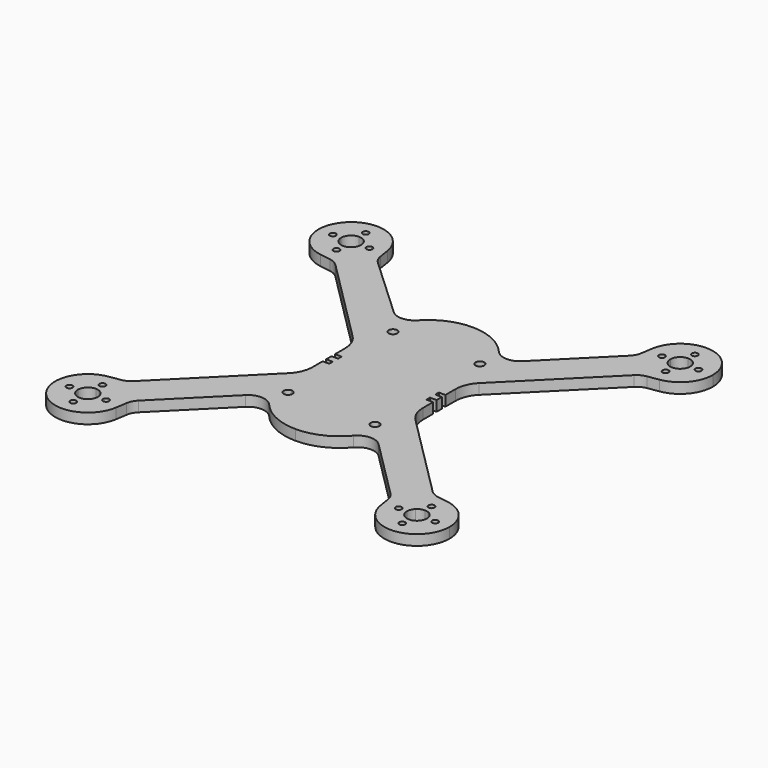
from build123d import *

# Parameters (mm, degrees)
F0_W     = 20
F0_H     = 20
F1_DEPTH = 2.38125


with BuildPart() as f1:
    # F0 (on Top) → F1 (new body)
    with BuildSketch(Plane.XY):
        with BuildLine():
            ThreePointArc((14.5598719395, -9.1717182668), (13.1833649686, -7.1116300018), (12.7, -4.6815902063))
            Line((12.7, -4.6815902063), (12.7, -1.778))
            Line((12.7, -1.778), (11.176, -1.778))
            Line((11.176, -1.778), (11.176, -0.762))
            Line((11.176, -0.762), (12.7, -0.762))
            Line((12.7, -0.762), (12.7, 0))
            Line((12.7, 0), (12.7, 0.762))
            Line((12.7, 0.762), (11.176, 0.762))
            Line((11.176, 0.762), (11.176, 1.778))
            Line((11.176, 1.778), (12.7, 1.778))
            Line((12.7, 1.778), (12.7, 4.6815902063))
            ThreePointArc((12.7, 4.6815902063), (13.1833649686, 7.1116300018), (14.5598719395, 9.1717182668))
            Line((14.5598719395, 9.1717182668), (34.3565237507, 28.9683700781))
            ThreePointArc((34.3565237507, 28.9683700781), (35.3250117586, 29.6711216441), (36.4637071746, 30.0388192574))
            Line((36.4637071746, 30.0388192574), (39.0000191321, 30.4342328562))
            ThreePointArc((39.0000191321, 30.4342328562), (35.5184477773, 30.7146069816), (32.5414162801, 32.5414162801))
            ThreePointArc((32.5414162801, 32.5414162801), (30.7146069816, 35.5184477773), (30.4342328562, 39.0000191321))
            Line((30.4342328562, 39.0000191321), (30.0388192574, 36.4637071746))
            ThreePointArc((30.0388192574, 36.4637071746), (29.6711216441, 35.3250117586), (28.9683700781, 34.3565237507))
            Line((28.9683700781, 34.3565237507), (15.290565472, 20.6787191446))
            ThreePointArc((15.290565472, 20.6787191446), (12.4394024333, 19.5660356884), (9.6896066428, 20.9098430623))
            ThreePointArc((9.6896066428, 20.9098430623), (5.3397094073, 24.2229121079), (0, 25.4))
            ThreePointArc((0, 25.4), (-5.0707891759, 24.3437578613), (-9.2981167449, 21.350723958))
            ThreePointArc((-9.2981167449, 21.350723958), (-11.9482165642, 20.1384898061), (-14.6798334501, 21.1537778832))
            Line((-14.6798334501, 21.1537778832), (-28.8786970448, 34.3361925702))
            ThreePointArc((-28.8786970448, 34.3361925702), (-29.650647044, 35.3400479178), (-30.0509413788, 36.5414624199))
            Line((-30.0509413788, 36.5414624199), (-30.4342328562, 39.0000191321))
            ThreePointArc((-30.4342328562, 39.0000191321), (-30.3671295561, 38.4240995168), (-30.344717139, 37.844717139))
            ThreePointArc((-30.344717139, 37.844717139), (-30.9156206452, 34.9745913963), (-32.5414162801, 32.5414162801))
            ThreePointArc((-32.5414162801, 32.5414162801), (-35.5184477773, 30.7146069816), (-39.0000191321, 30.4342328562))
            Line((-39.0000191321, 30.4342328562), (-36.4637071746, 30.0388192574))
            ThreePointArc((-36.4637071746, 30.0388192574), (-35.3250117586, 29.6711216441), (-34.3565237507, 28.9683700781))
            Line((-34.3565237507, 28.9683700781), (-14.5598719395, 9.1717182668))
            ThreePointArc((-14.5598719395, 9.1717182668), (-13.1833649686, 7.1116300018), (-12.7, 4.6815902063))
            Line((-12.7, 4.6815902063), (-12.7, 1.778))
            Line((-12.7, 1.778), (-11.176, 1.778))
            Line((-11.176, 1.778), (-11.176, 0.762))
            Line((-11.176, 0.762), (-12.7, 0.762))
            Line((-12.7, 0.762), (-12.7, 0))
            Line((-12.7, 0), (-12.7, -0.762))
            Line((-12.7, -0.762), (-11.176, -0.762))
            Line((-11.176, -0.762), (-11.176, -1.778))
            Line((-11.176, -1.778), (-12.7, -1.778))
            Line((-12.7, -1.778), (-12.7, -4.6815902063))
            ThreePointArc((-12.7, -4.6815902063), (-13.1833649686, -7.1116300018), (-14.5598719395, -9.1717182668))
            Line((-14.5598719395, -9.1717182668), (-34.3565237507, -28.9683700781))
            ThreePointArc((-34.3565237507, -28.9683700781), (-35.3250117586, -29.6711216441), (-36.4637071746, -30.0388192574))
            Line((-36.4637071746, -30.0388192574), (-39.0000191321, -30.4342328562))
            ThreePointArc((-39.0000191321, -30.4342328562), (-35.5184477773, -30.7146069816), (-32.5414162801, -32.5414162801))
            ThreePointArc((-32.5414162801, -32.5414162801), (-30.9156206452, -34.9745913963), (-30.344717139, -37.844717139))
            ThreePointArc((-30.344717139, -37.844717139), (-30.3671295561, -38.4240995168), (-30.4342328562, -39.0000191321))
            Line((-30.4342328562, -39.0000191321), (-30.0388192574, -36.4637071746))
            ThreePointArc((-30.0388192574, -36.4637071746), (-29.6711216441, -35.3250117586), (-28.9683700781, -34.3565237507))
            Line((-28.9683700781, -34.3565237507), (-15.290565472, -20.6787191446))
            ThreePointArc((-15.290565472, -20.6787191446), (-12.4394024333, -19.5660356884), (-9.6896066428, -20.9098430623))
            ThreePointArc((-9.6896066428, -20.9098430623), (-5.3397094073, -24.2229121079), (0, -25.4))
            ThreePointArc((0, -25.4), (5.3397094073, -24.2229121079), (9.6896066428, -20.9098430623))
            ThreePointArc((9.6896066428, -20.9098430623), (12.4394024333, -19.5660356884), (15.290565472, -20.6787191446))
            Line((15.290565472, -20.6787191446), (28.9683700781, -34.3565237507))
            ThreePointArc((28.9683700781, -34.3565237507), (29.6711216441, -35.3250117586), (30.0388192574, -36.4637071746))
            Line((30.0388192574, -36.4637071746), (30.4342328562, -39.0000191321))
            ThreePointArc((30.4342328562, -39.0000191321), (30.7146069816, -35.5184477773), (32.5414162801, -32.5414162801))
            ThreePointArc((32.5414162801, -32.5414162801), (35.5184477773, -30.7146069816), (39.0000191321, -30.4342328562))
            Line((39.0000191321, -30.4342328562), (36.4637071746, -30.0388192574))
            ThreePointArc((36.4637071746, -30.0388192574), (35.3250117586, -29.6711216441), (34.3565237507, -28.9683700781))
            Line((34.3565237507, -28.9683700781), (14.5598719395, -9.1717182668))
        make_face()
        with BuildLine():
            ThreePointArc((-9, -15.08), (-10.7071067812, -15.7871067812), (-10, -14.08))
            ThreePointArc((-10, -14.08), (-9.2928932188, -14.3728932188), (-9, -15.08))
        make_face(mode=Mode.SUBTRACT)
        with BuildLine():
            ThreePointArc((11, -15.08), (9.2928932188, -15.7871067812), (10, -14.08))
            ThreePointArc((10, -14.08), (10.7071067812, -14.3728932188), (11, -15.08))
        make_face(mode=Mode.SUBTRACT)
        with BuildLine():
            ThreePointArc((-9, 15.08), (-9.2928932188, 14.3728932188), (-10, 14.08))
            ThreePointArc((-10, 14.08), (-10.7071067812, 15.7871067812), (-9, 15.08))
        make_face(mode=Mode.SUBTRACT)
        Rectangle(F0_W, F0_H, mode=Mode.SUBTRACT)
        with BuildLine():
            ThreePointArc((11, 15.08), (10.7071067812, 14.3728932188), (10, 14.08))
            ThreePointArc((10, 14.08), (9.2928932188, 15.7871067812), (11, 15.08))
        make_face(mode=Mode.SUBTRACT)
        Rectangle(F0_W, F0_H)
        with BuildLine():
            ThreePointArc((45.344717139, -37.844717139), (43.541855234, -32.9669494604), (39.0000191321, -30.4342328562))
            ThreePointArc((39.0000191321, -30.4342328562), (35.5184477773, -30.7146069816), (32.5414162801, -32.5414162801))
            ThreePointArc((32.5414162801, -32.5414162801), (30.7146069816, -35.5184477773), (30.4342328562, -39.0000191321))
            ThreePointArc((30.4342328562, -39.0000191321), (38.4240995168, -45.3223047219), (45.344717139, -37.844717139))
        make_face()
        with BuildLine():
            ThreePointArc((33.7030504723, -37.147151929), (34.1118590196, -35.9196794094), (34.874868658, -34.874868658))
            ThreePointArc((34.874868658, -34.874868658), (35.9196794094, -34.1118590196), (37.147151929, -33.7030504723))
            ThreePointArc((37.147151929, -33.7030504723), (37.8155250768, -32.9453261014), (38.544717139, -33.644717139))
            ThreePointArc((38.544717139, -33.644717139), (38.5441081766, -33.6739092012), (38.542282349, -33.7030504723))
            ThreePointArc((38.542282349, -33.7030504723), (40.81456562, -34.874868658), (41.9863838057, -37.147151929))
            ThreePointArc((41.9863838057, -37.147151929), (42.5186193793, -37.3295310885), (42.744717139, -37.844717139))
            ThreePointArc((42.744717139, -37.844717139), (42.5186193793, -38.3599031895), (41.9863838057, -38.542282349))
            ThreePointArc((41.9863838057, -38.542282349), (40.81456562, -40.81456562), (38.542282349, -41.9863838057))
            ThreePointArc((38.542282349, -41.9863838057), (38.5441081766, -42.0155250768), (38.544717139, -42.044717139))
            ThreePointArc((38.544717139, -42.044717139), (37.8155250768, -42.7441081766), (37.147151929, -41.9863838057))
            ThreePointArc((37.147151929, -41.9863838057), (34.874868658, -40.81456562), (33.7030504723, -38.542282349))
            ThreePointArc((33.7030504723, -38.542282349), (32.944717139, -37.844717139), (33.7030504723, -37.147151929))
        make_face(mode=Mode.SUBTRACT)
        with BuildLine():
            ThreePointArc((32.5414162801, 32.5414162801), (35.5184477773, 30.7146069816), (39.0000191321, 30.4342328562))
            ThreePointArc((39.0000191321, 30.4342328562), (43.541855234, 32.9669494604), (45.344717139, 37.844717139))
            ThreePointArc((45.344717139, 37.844717139), (38.4240995168, 45.3223047219), (30.4342328562, 39.0000191321))
            ThreePointArc((30.4342328562, 39.0000191321), (30.7146069816, 35.5184477773), (32.5414162801, 32.5414162801))
        make_face()
        with BuildLine():
            ThreePointArc((37.147151929, 33.7030504723), (35.9196794094, 34.1118590196), (34.874868658, 34.874868658))
            ThreePointArc((34.874868658, 34.874868658), (34.1118590196, 35.9196794094), (33.7030504723, 37.147151929))
            ThreePointArc((33.7030504723, 37.147151929), (32.944717139, 37.844717139), (33.7030504723, 38.542282349))
            ThreePointArc((33.7030504723, 38.542282349), (34.874868658, 40.81456562), (37.147151929, 41.9863838057))
            ThreePointArc((37.147151929, 41.9863838057), (37.8155250768, 42.7441081766), (38.544717139, 42.044717139))
            ThreePointArc((38.544717139, 42.044717139), (38.5441081766, 42.0155250768), (38.542282349, 41.9863838057))
            ThreePointArc((38.542282349, 41.9863838057), (40.81456562, 40.81456562), (41.9863838057, 38.542282349))
            ThreePointArc((41.9863838057, 38.542282349), (42.5186193793, 38.3599031895), (42.744717139, 37.844717139))
            ThreePointArc((42.744717139, 37.844717139), (42.5186193793, 37.3295310885), (41.9863838057, 37.147151929))
            ThreePointArc((41.9863838057, 37.147151929), (40.81456562, 34.874868658), (38.542282349, 33.7030504723))
            ThreePointArc((38.542282349, 33.7030504723), (38.5441081766, 33.6739092012), (38.544717139, 33.644717139))
            ThreePointArc((38.544717139, 33.644717139), (37.8155250768, 32.9453261014), (37.147151929, 33.7030504723))
        make_face(mode=Mode.SUBTRACT)
        with BuildLine():
            ThreePointArc((-39.0000191321, -30.4342328562), (-43.1480179979, -43.1480179979), (-30.4342328562, -39.0000191321))
            ThreePointArc((-30.4342328562, -39.0000191321), (-30.3671295561, -38.4240995168), (-30.344717139, -37.844717139))
            ThreePointArc((-30.344717139, -37.844717139), (-30.9156206452, -34.9745913963), (-32.5414162801, -32.5414162801))
            ThreePointArc((-32.5414162801, -32.5414162801), (-35.5184477773, -30.7146069816), (-39.0000191321, -30.4342328562))
        make_face()
        with BuildLine():
            ThreePointArc((-37.147151929, -33.7030504723), (-35.9196794094, -34.1118590196), (-34.874868658, -34.874868658))
            ThreePointArc((-34.874868658, -34.874868658), (-34.1118590196, -35.9196794094), (-33.7030504723, -37.147151929))
            ThreePointArc((-33.7030504723, -37.147151929), (-33.1708148987, -37.3295310885), (-32.944717139, -37.844717139))
            ThreePointArc((-32.944717139, -37.844717139), (-33.1708148987, -38.3599031895), (-33.7030504723, -38.542282349))
            ThreePointArc((-33.7030504723, -38.542282349), (-34.874868658, -40.81456562), (-37.147151929, -41.9863838057))
            ThreePointArc((-37.147151929, -41.9863838057), (-37.1453261014, -42.0155250768), (-37.144717139, -42.044717139))
            ThreePointArc((-37.144717139, -42.044717139), (-37.8739092012, -42.7441081766), (-38.542282349, -41.9863838057))
            ThreePointArc((-38.542282349, -41.9863838057), (-40.81456562, -40.81456562), (-41.9863838057, -38.542282349))
            ThreePointArc((-41.9863838057, -38.542282349), (-42.744717139, -37.844717139), (-41.9863838057, -37.147151929))
            ThreePointArc((-41.9863838057, -37.147151929), (-40.81456562, -34.874868658), (-38.542282349, -33.7030504723))
            ThreePointArc((-38.542282349, -33.7030504723), (-37.8739092012, -32.9453261014), (-37.144717139, -33.644717139))
            ThreePointArc((-37.144717139, -33.644717139), (-37.1453261014, -33.6739092012), (-37.147151929, -33.7030504723))
        make_face(mode=Mode.SUBTRACT)
        with BuildLine():
            ThreePointArc((-30.344717139, 37.844717139), (-30.3671295561, 38.4240995168), (-30.4342328562, 39.0000191321))
            ThreePointArc((-30.4342328562, 39.0000191321), (-43.1480179979, 43.1480179979), (-39.0000191321, 30.4342328562))
            ThreePointArc((-39.0000191321, 30.4342328562), (-35.5184477773, 30.7146069816), (-32.5414162801, 32.5414162801))
            ThreePointArc((-32.5414162801, 32.5414162801), (-30.9156206452, 34.9745913963), (-30.344717139, 37.844717139))
        make_face()
        with BuildLine():
            ThreePointArc((-33.7030504723, 37.147151929), (-34.1118590196, 35.9196794094), (-34.874868658, 34.874868658))
            ThreePointArc((-34.874868658, 34.874868658), (-35.9196794094, 34.1118590196), (-37.147151929, 33.7030504723))
            ThreePointArc((-37.147151929, 33.7030504723), (-37.1453261014, 33.6739092012), (-37.144717139, 33.644717139))
            ThreePointArc((-37.144717139, 33.644717139), (-37.8739092012, 32.9453261014), (-38.542282349, 33.7030504723))
            ThreePointArc((-38.542282349, 33.7030504723), (-40.81456562, 34.874868658), (-41.9863838057, 37.147151929))
            ThreePointArc((-41.9863838057, 37.147151929), (-42.744717139, 37.844717139), (-41.9863838057, 38.542282349))
            ThreePointArc((-41.9863838057, 38.542282349), (-40.81456562, 40.81456562), (-38.542282349, 41.9863838057))
            ThreePointArc((-38.542282349, 41.9863838057), (-37.8739092012, 42.7441081766), (-37.144717139, 42.044717139))
            ThreePointArc((-37.144717139, 42.044717139), (-37.1453261014, 42.0155250768), (-37.147151929, 41.9863838057))
            ThreePointArc((-37.147151929, 41.9863838057), (-34.874868658, 40.81456562), (-33.7030504723, 38.542282349))
            ThreePointArc((-33.7030504723, 38.542282349), (-33.1708148987, 38.3599031895), (-32.944717139, 37.844717139))
            ThreePointArc((-32.944717139, 37.844717139), (-33.1708148987, 37.3295310885), (-33.7030504723, 37.147151929))
        make_face(mode=Mode.SUBTRACT)
        with BuildLine():
            Line((37.844717139, -34.344717139), (37.844717139, -35.558717139))
            ThreePointArc((37.844717139, -35.558717139), (39.4611632408, -36.2282710372), (40.130717139, -37.844717139))
            Line((40.130717139, -37.844717139), (41.344717139, -37.844717139))
            ThreePointArc((41.344717139, -37.844717139), (41.5295310885, -37.3708148987), (41.9863838057, -37.147151929))
            ThreePointArc((41.9863838057, -37.147151929), (40.81456562, -34.874868658), (38.542282349, -33.7030504723))
            ThreePointArc((38.542282349, -33.7030504723), (38.3186193793, -34.1599031895), (37.844717139, -34.344717139))
        make_face()
        with BuildLine():
            ThreePointArc((37.844717139, -40.130717139), (36.2282710372, -39.4611632408), (35.558717139, -37.844717139))
            Line((35.558717139, -37.844717139), (34.344717139, -37.844717139))
            ThreePointArc((34.344717139, -37.844717139), (34.1599031895, -38.3186193793), (33.7030504723, -38.542282349))
            ThreePointArc((33.7030504723, -38.542282349), (34.874868658, -40.81456562), (37.147151929, -41.9863838057))
            ThreePointArc((37.147151929, -41.9863838057), (37.3708148987, -41.5295310885), (37.844717139, -41.344717139))
            Line((37.844717139, -41.344717139), (37.844717139, -40.130717139))
        make_face()
        with BuildLine():
            Line((41.344717139, -37.844717139), (40.130717139, -37.844717139))
            ThreePointArc((40.130717139, -37.844717139), (39.4611632408, -39.4611632408), (37.844717139, -40.130717139))
            Line((37.844717139, -40.130717139), (37.844717139, -41.344717139))
            ThreePointArc((37.844717139, -41.344717139), (38.3186193793, -41.5295310885), (38.542282349, -41.9863838057))
            ThreePointArc((38.542282349, -41.9863838057), (40.81456562, -40.81456562), (41.9863838057, -38.542282349))
            ThreePointArc((41.9863838057, -38.542282349), (41.5295310885, -38.3186193793), (41.344717139, -37.844717139))
        make_face()
        with BuildLine():
            Line((34.344717139, 37.844717139), (35.558717139, 37.844717139))
            ThreePointArc((35.558717139, 37.844717139), (36.2282710372, 39.4611632408), (37.844717139, 40.130717139))
            Line((37.844717139, 40.130717139), (37.844717139, 41.344717139))
            ThreePointArc((37.844717139, 41.344717139), (37.3708148987, 41.5295310885), (37.147151929, 41.9863838057))
            ThreePointArc((37.147151929, 41.9863838057), (34.874868658, 40.81456562), (33.7030504723, 38.542282349))
            ThreePointArc((33.7030504723, 38.542282349), (34.1599031895, 38.3186193793), (34.344717139, 37.844717139))
        make_face()
        with BuildLine():
            ThreePointArc((40.130717139, 37.844717139), (39.4611632408, 36.2282710372), (37.844717139, 35.558717139))
            Line((37.844717139, 35.558717139), (37.844717139, 34.344717139))
            ThreePointArc((37.844717139, 34.344717139), (38.3186193793, 34.1599031895), (38.542282349, 33.7030504723))
            ThreePointArc((38.542282349, 33.7030504723), (40.81456562, 34.874868658), (41.9863838057, 37.147151929))
            ThreePointArc((41.9863838057, 37.147151929), (41.5295310885, 37.3708148987), (41.344717139, 37.844717139))
            Line((41.344717139, 37.844717139), (40.130717139, 37.844717139))
        make_face()
        with BuildLine():
            ThreePointArc((37.844717139, 40.130717139), (39.4611632408, 39.4611632408), (40.130717139, 37.844717139))
            Line((40.130717139, 37.844717139), (41.344717139, 37.844717139))
            ThreePointArc((41.344717139, 37.844717139), (41.5295310885, 38.3186193793), (41.9863838057, 38.542282349))
            ThreePointArc((41.9863838057, 38.542282349), (40.81456562, 40.81456562), (38.542282349, 41.9863838057))
            ThreePointArc((38.542282349, 41.9863838057), (38.3186193793, 41.5295310885), (37.844717139, 41.344717139))
            Line((37.844717139, 41.344717139), (37.844717139, 40.130717139))
        make_face()
        with BuildLine():
            Line((-34.344717139, -37.844717139), (-35.558717139, -37.844717139))
            ThreePointArc((-35.558717139, -37.844717139), (-36.2282710372, -39.4611632408), (-37.844717139, -40.130717139))
            Line((-37.844717139, -40.130717139), (-37.844717139, -41.344717139))
            ThreePointArc((-37.844717139, -41.344717139), (-37.3708148987, -41.5295310885), (-37.147151929, -41.9863838057))
            ThreePointArc((-37.147151929, -41.9863838057), (-34.874868658, -40.81456562), (-33.7030504723, -38.542282349))
            ThreePointArc((-33.7030504723, -38.542282349), (-34.1599031895, -38.3186193793), (-34.344717139, -37.844717139))
        make_face()
        with BuildLine():
            ThreePointArc((-40.130717139, -37.844717139), (-39.4611632408, -36.2282710372), (-37.844717139, -35.558717139))
            Line((-37.844717139, -35.558717139), (-37.844717139, -34.344717139))
            ThreePointArc((-37.844717139, -34.344717139), (-38.3186193793, -34.1599031895), (-38.542282349, -33.7030504723))
            ThreePointArc((-38.542282349, -33.7030504723), (-40.81456562, -34.874868658), (-41.9863838057, -37.147151929))
            ThreePointArc((-41.9863838057, -37.147151929), (-41.5295310885, -37.3708148987), (-41.344717139, -37.844717139))
            Line((-41.344717139, -37.844717139), (-40.130717139, -37.844717139))
        make_face()
        with BuildLine():
            Line((-37.844717139, -41.344717139), (-37.844717139, -40.130717139))
            ThreePointArc((-37.844717139, -40.130717139), (-39.4611632408, -39.4611632408), (-40.130717139, -37.844717139))
            Line((-40.130717139, -37.844717139), (-41.344717139, -37.844717139))
            ThreePointArc((-41.344717139, -37.844717139), (-41.5295310885, -38.3186193793), (-41.9863838057, -38.542282349))
            ThreePointArc((-41.9863838057, -38.542282349), (-40.81456562, -40.81456562), (-38.542282349, -41.9863838057))
            ThreePointArc((-38.542282349, -41.9863838057), (-38.3186193793, -41.5295310885), (-37.844717139, -41.344717139))
        make_face()
        with BuildLine():
            Line((-37.844717139, 34.344717139), (-37.844717139, 35.558717139))
            ThreePointArc((-37.844717139, 35.558717139), (-39.4611632408, 36.2282710372), (-40.130717139, 37.844717139))
            Line((-40.130717139, 37.844717139), (-41.344717139, 37.844717139))
            ThreePointArc((-41.344717139, 37.844717139), (-41.5295310885, 37.3708148987), (-41.9863838057, 37.147151929))
            ThreePointArc((-41.9863838057, 37.147151929), (-40.81456562, 34.874868658), (-38.542282349, 33.7030504723))
            ThreePointArc((-38.542282349, 33.7030504723), (-38.3186193793, 34.1599031895), (-37.844717139, 34.344717139))
        make_face()
        with BuildLine():
            ThreePointArc((-37.844717139, 40.130717139), (-36.2282710372, 39.4611632408), (-35.558717139, 37.844717139))
            Line((-35.558717139, 37.844717139), (-34.344717139, 37.844717139))
            ThreePointArc((-34.344717139, 37.844717139), (-34.1599031895, 38.3186193793), (-33.7030504723, 38.542282349))
            ThreePointArc((-33.7030504723, 38.542282349), (-34.874868658, 40.81456562), (-37.147151929, 41.9863838057))
            ThreePointArc((-37.147151929, 41.9863838057), (-37.3708148987, 41.5295310885), (-37.844717139, 41.344717139))
            Line((-37.844717139, 41.344717139), (-37.844717139, 40.130717139))
        make_face()
        with BuildLine():
            ThreePointArc((-40.130717139, 37.844717139), (-39.4611632408, 39.4611632408), (-37.844717139, 40.130717139))
            Line((-37.844717139, 40.130717139), (-37.844717139, 41.344717139))
            ThreePointArc((-37.844717139, 41.344717139), (-38.3186193793, 41.5295310885), (-38.542282349, 41.9863838057))
            ThreePointArc((-38.542282349, 41.9863838057), (-40.81456562, 40.81456562), (-41.9863838057, 38.542282349))
            ThreePointArc((-41.9863838057, 38.542282349), (-41.5295310885, 38.3186193793), (-41.344717139, 37.844717139))
            Line((-41.344717139, 37.844717139), (-40.130717139, 37.844717139))
        make_face()
        with BuildLine():
            ThreePointArc((37.147151929, -33.7030504723), (35.9196794094, -34.1118590196), (34.874868658, -34.874868658))
            Line((34.874868658, -34.874868658), (36.2282710372, -36.2282710372))
            ThreePointArc((36.2282710372, -36.2282710372), (36.9699028126, -35.7327285277), (37.844717139, -35.558717139))
            Line((37.844717139, -35.558717139), (37.844717139, -34.344717139))
            ThreePointArc((37.844717139, -34.344717139), (37.3708148987, -34.1599031895), (37.147151929, -33.7030504723))
        make_face()
        with BuildLine():
            Line((36.2282710372, -36.2282710372), (34.874868658, -34.874868658))
            ThreePointArc((34.874868658, -34.874868658), (34.1118590196, -35.9196794094), (33.7030504723, -37.147151929))
            ThreePointArc((33.7030504723, -37.147151929), (34.1599031895, -37.3708148987), (34.344717139, -37.844717139))
            Line((34.344717139, -37.844717139), (35.558717139, -37.844717139))
            ThreePointArc((35.558717139, -37.844717139), (35.7327285277, -36.9699028126), (36.2282710372, -36.2282710372))
        make_face()
        with BuildLine():
            ThreePointArc((33.7030504723, 37.147151929), (34.1118590196, 35.9196794094), (34.874868658, 34.874868658))
            Line((34.874868658, 34.874868658), (36.2282710372, 36.2282710372))
            ThreePointArc((36.2282710372, 36.2282710372), (35.7327285277, 36.9699028126), (35.558717139, 37.844717139))
            Line((35.558717139, 37.844717139), (34.344717139, 37.844717139))
            ThreePointArc((34.344717139, 37.844717139), (34.1599031895, 37.3708148987), (33.7030504723, 37.147151929))
        make_face()
        with BuildLine():
            Line((36.2282710372, 36.2282710372), (34.874868658, 34.874868658))
            ThreePointArc((34.874868658, 34.874868658), (35.9196794094, 34.1118590196), (37.147151929, 33.7030504723))
            ThreePointArc((37.147151929, 33.7030504723), (37.3708148987, 34.1599031895), (37.844717139, 34.344717139))
            Line((37.844717139, 34.344717139), (37.844717139, 35.558717139))
            ThreePointArc((37.844717139, 35.558717139), (36.9699028126, 35.7327285277), (36.2282710372, 36.2282710372))
        make_face()
        with BuildLine():
            ThreePointArc((-33.7030504723, -37.147151929), (-34.1118590196, -35.9196794094), (-34.874868658, -34.874868658))
            Line((-34.874868658, -34.874868658), (-36.2282710372, -36.2282710372))
            ThreePointArc((-36.2282710372, -36.2282710372), (-35.7327285277, -36.9699028126), (-35.558717139, -37.844717139))
            Line((-35.558717139, -37.844717139), (-34.344717139, -37.844717139))
            ThreePointArc((-34.344717139, -37.844717139), (-34.1599031895, -37.3708148987), (-33.7030504723, -37.147151929))
        make_face()
        with BuildLine():
            Line((-36.2282710372, -36.2282710372), (-34.874868658, -34.874868658))
            ThreePointArc((-34.874868658, -34.874868658), (-35.9196794094, -34.1118590196), (-37.147151929, -33.7030504723))
            ThreePointArc((-37.147151929, -33.7030504723), (-37.3708148987, -34.1599031895), (-37.844717139, -34.344717139))
            Line((-37.844717139, -34.344717139), (-37.844717139, -35.558717139))
            ThreePointArc((-37.844717139, -35.558717139), (-36.9699028126, -35.7327285277), (-36.2282710372, -36.2282710372))
        make_face()
        with BuildLine():
            ThreePointArc((-37.147151929, 33.7030504723), (-35.9196794094, 34.1118590196), (-34.874868658, 34.874868658))
            Line((-34.874868658, 34.874868658), (-36.2282710372, 36.2282710372))
            ThreePointArc((-36.2282710372, 36.2282710372), (-36.9699028126, 35.7327285277), (-37.844717139, 35.558717139))
            Line((-37.844717139, 35.558717139), (-37.844717139, 34.344717139))
            ThreePointArc((-37.844717139, 34.344717139), (-37.3708148987, 34.1599031895), (-37.147151929, 33.7030504723))
        make_face()
        with BuildLine():
            Line((-36.2282710372, 36.2282710372), (-34.874868658, 34.874868658))
            ThreePointArc((-34.874868658, 34.874868658), (-34.1118590196, 35.9196794094), (-33.7030504723, 37.147151929))
            ThreePointArc((-33.7030504723, 37.147151929), (-34.1599031895, 37.3708148987), (-34.344717139, 37.844717139))
            Line((-34.344717139, 37.844717139), (-35.558717139, 37.844717139))
            ThreePointArc((-35.558717139, 37.844717139), (-35.7327285277, 36.9699028126), (-36.2282710372, 36.2282710372))
        make_face()
    extrude(amount=F1_DEPTH)


solid = f1.part
